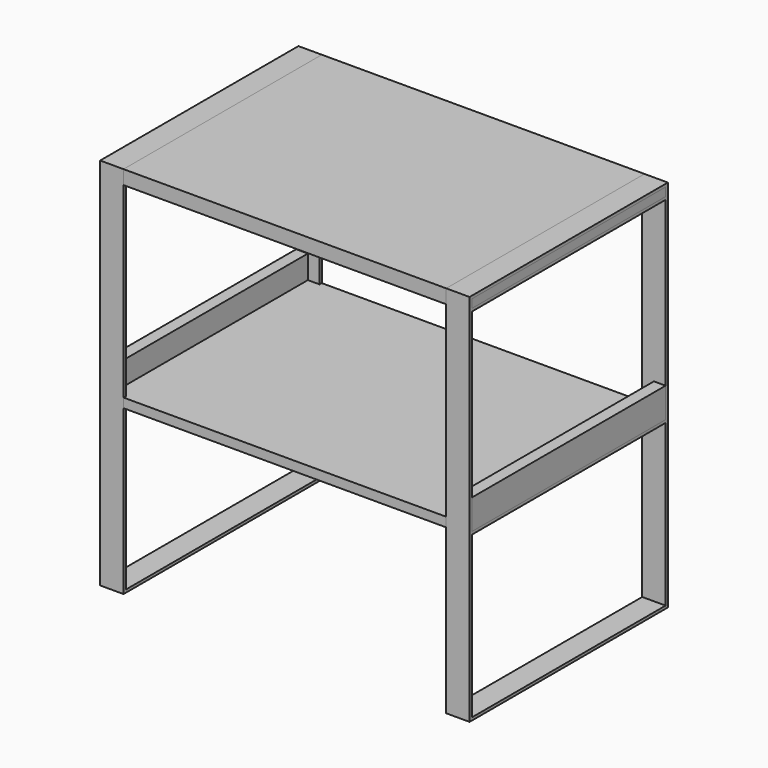
from build123d import *

# Parameters (mm, degrees)
F2_W           = 50
F2_H           = 6
F3_DEPTH       = 800
F4_W           = 50
F4_H           = 6
F5_DEPTH       = 518
F10_W          = 530
F10_H          = 30
F11_DEPTH      = 395
F11_DEPTH_BACK = 395
F10_H_2        = 20
F14_W          = 25
F14_H          = 530
F15_DEPTH      = 50


with BuildPart() as f3:
    # F2 (on Top) → F3 (new body)
    with BuildSketch(Plane.XY):
        with Locations((-370, -262)):
            Rectangle(F2_W, F2_H)
    extrude(amount=F3_DEPTH)



with BuildPart() as f3b:
    # F2 (on Top) → F3, piece 2 (new body)
    with BuildSketch(Plane.XY):
        with Locations((-370, 262)):
            Rectangle(F2_W, F2_H)
    extrude(amount=F3_DEPTH)


with BuildPart() as f3c:
    # F2 (on Top) → F3, piece 3 (new body)
    with BuildSketch(Plane.XY):
        with Locations((370, -262)):
            Rectangle(F2_W, F2_H)
    extrude(amount=F3_DEPTH)



with BuildPart() as f3d:
    # F2 (on Top) → F3, piece 4 (new body)
    with BuildSketch(Plane.XY):
        with Locations((370, 262)):
            Rectangle(F2_W, F2_H)
    extrude(amount=F3_DEPTH)


with BuildPart() as f3c_1:
    add(f3c.part)

    add(f3d.part)  # F5 merges F3d
    # F4 (on face) → F5 (join, through all)
    with BuildSketch(Plane(origin=(0, -259, 0), x_dir=(-1, 0, 0), z_dir=(0, 1, 0))):
        with Locations((-370, 797)):
            Rectangle(F4_W, F4_H)
        with Locations((-370, 773)):
            Rectangle(F4_W, F4_H)
        with Locations((-370, 3)):
            Rectangle(F4_W, F4_H)
        with Locations((-370, 353)):
            Rectangle(F4_W, F4_H)
    extrude(amount=F5_DEPTH)

    # F6: union 

    # F8: union 


with BuildPart() as f3_1:
    add(f3.part)

    add(f3b.part)  # F5#2 merges F3b
    # F4 (on face) → F5, piece 2 (join, through all)
    with BuildSketch(Plane(origin=(0, -259, 0), x_dir=(-1, 0, 0), z_dir=(0, 1, 0))):
        with Locations((370, 773)):
            Rectangle(F4_W, F4_H)
        with Locations((370, 797)):
            Rectangle(F4_W, F4_H)
        with Locations((370, 3)):
            Rectangle(F4_W, F4_H)
        with Locations((370, 353)):
            Rectangle(F4_W, F4_H)
    extrude(amount=F5_DEPTH)

    # F7: union 

    # F9: union 


with BuildPart() as f11:
    # F10 (on Right) → F11 (new body, two sides)
    with BuildSketch(Plane.YZ) as f11_sk:
        with Locations((0, 785)):
            Rectangle(F10_W, F10_H)
    extrude(amount=F11_DEPTH)
    extrude(f11_sk.sketch, amount=-F11_DEPTH_BACK)

    # F13: cut F3, F3c
    add(f3_1.part, mode=Mode.SUBTRACT)
    add(f3c_1.part, mode=Mode.SUBTRACT)


with BuildPart() as f11b:
    # F10 (on Right) → F11, piece 2 (new body, two sides)
    with BuildSketch(Plane.YZ) as f11_2_sk:
        with Locations((0, 360)):
            Rectangle(F10_W, F10_H_2)
    extrude(amount=F11_DEPTH)
    extrude(f11_2_sk.sketch, amount=-F11_DEPTH_BACK)

    # F12: cut F3, F3c
    add(f3_1.part, mode=Mode.SUBTRACT)
    add(f3c_1.part, mode=Mode.SUBTRACT)

    # F14 (on face) → F15 (join)
    with BuildSketch(Plane.XY.offset(370)):
        with Locations((382.5, 0)):
            Rectangle(F14_W, F14_H)
        with Locations((-382.5, 0)):
            Rectangle(F14_W, F14_H)
    extrude(amount=F15_DEPTH)

    # F16: cut F3c, F3
    add(f3c_1.part, mode=Mode.SUBTRACT)
    add(f3_1.part, mode=Mode.SUBTRACT)


solid = Compound([f3c_1.part, f3_1.part, f11.part, f11b.part])
